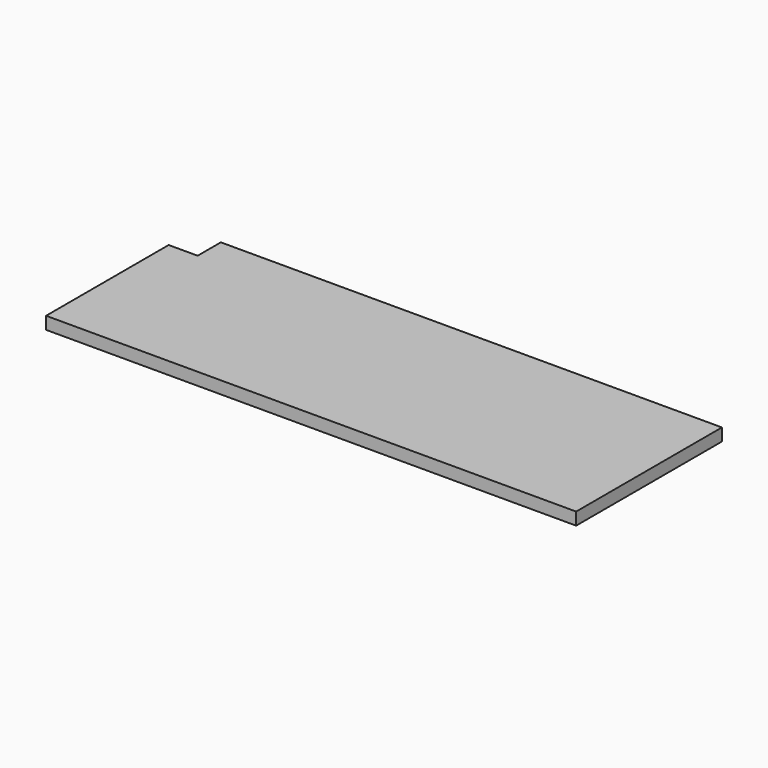
from build123d import *

# Parameters (mm, degrees)
F0_W     = 1625.6
F0_H     = 558.8
F1_DEPTH = 38.1
F2_W     = 88.9
F2_H     = 88.9
F3_DEPTH = 38.101


# Not quite as in the source:
# - a feature names something its author has since deleted; it is built from what else it names


with BuildPart() as f1:
    # F0 (on Top) → F1 (new body)
    with BuildSketch(Plane.XY):
        Rectangle(F0_W, F0_H)
    extrude(amount=F1_DEPTH)

    # F2 (on face) → F3 (cut, through all)
    with BuildSketch(Plane.XY.offset(38.1)):
        with Locations((-768.35, 234.95)):
            Rectangle(F2_W, F2_H)
    extrude(amount=-F3_DEPTH, mode=Mode.SUBTRACT)


solid = f1.part
